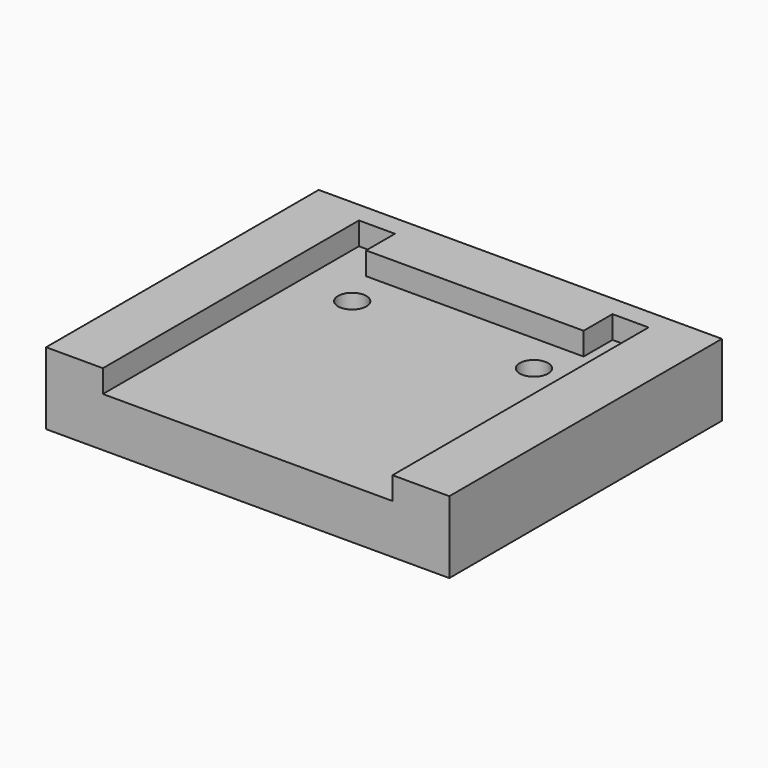
from build123d import *

# Parameters (mm, degrees)
F0_R     = 2.5
F1_DEPTH = 12.7
F2_DEPTH = 4


# Not quite as in the source:
# - a length typed as a fraction of an inch, garbled in the dataset ("3 / 203.2 mm" for 3/8 in), is restored
# - a feature names something its author has since deleted; it is built from what else it names


with BuildPart() as f1:
    # F0 (on Top) → F1 (new body)
    with BuildSketch(Plane.XY):
        Polygon((0, 60), (0, 0), (10, 0), (10, 50), (10, 56.35), (16.35, 56.35), (16.35, 50), (54.65, 50), (54.65, 56.35), (61, 56.35), (61, 50), (61, 0), (71, 0), (71, 60), align=None)
        Polygon((10, 50), (10, 0), (61, 0), (61, 50), (61, 56.35), (54.65, 56.35), (54.65, 50), (16.35, 50), (16.35, 56.35), (10, 56.35), align=None)
        with Locations((19.5, 43)):
            Circle(F0_R, mode=Mode.SUBTRACT)
        with Locations((51.5, 43)):
            Circle(F0_R, mode=Mode.SUBTRACT)
    extrude(amount=-F1_DEPTH)

    # F0 (on Top) → F2 (cut)
    with BuildSketch(Plane.XY):
        Polygon((10, 50), (10, 0), (61, 0), (61, 50), (61, 56.35), (54.65, 56.35), (54.65, 50), (16.35, 50), (16.35, 56.35), (10, 56.35), align=None)
        with Locations((19.5, 43)):
            Circle(F0_R, mode=Mode.SUBTRACT)
        with Locations((51.5, 43)):
            Circle(F0_R, mode=Mode.SUBTRACT)
    extrude(amount=-F2_DEPTH, mode=Mode.SUBTRACT)


solid = f1.part
